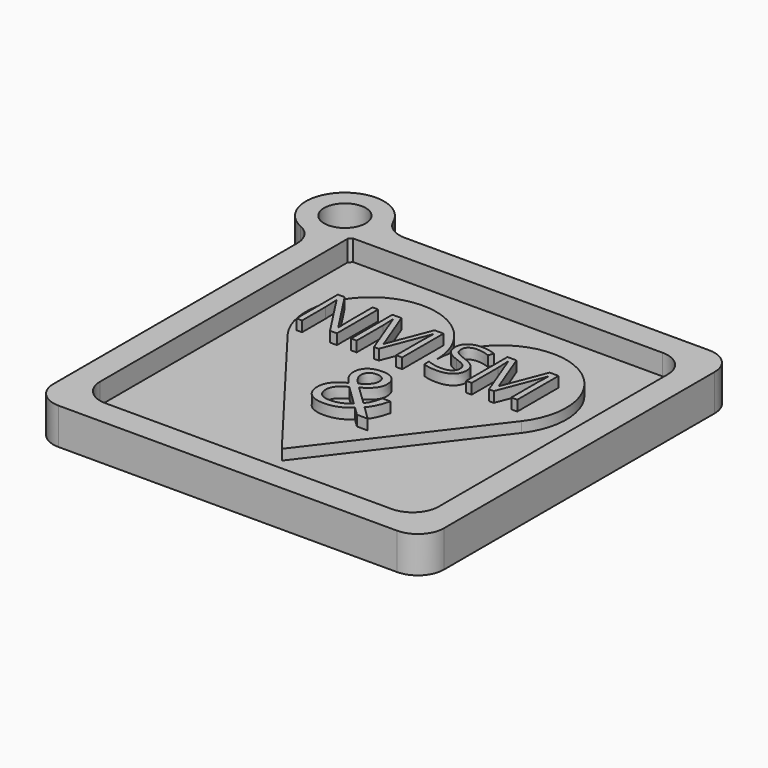
from build123d import *

# Parameters (mm, degrees)
F1_DEPTH       = 3
F2_DEPTH       = 5
F3_TEXT_SIZE   = 13.8888888889
F3_TEXT_SIZE_2 = 18.3928938996
F4_DEPTH       = 2
F5_DEPTH       = 2
F6_R           = 5


# Not quite as in the source:
# - a feature names something its author has since deleted; it is built from what else it names
# - Text() gives the source's letters only with a copy of the font that has no kerning and outlines rounded to 1/6400 em; it was checked with that copy


with BuildPart() as f1:
    # F0 (on Top) → F1 (new body)
    with BuildSketch(Plane.XY):
        with BuildLine():
            Line((32.5, 32.5), (-31.9098300563, 32.5))
            ThreePointArc((-31.9098300563, 32.5), (-32.1966991411, 32.1966991411), (-32.5, 31.9098300563))
            Line((-32.5, 31.9098300563), (-32.5, -32.5))
            Line((-32.5, -32.5), (32.5, -32.5))
            Line((32.5, -32.5), (32.5, 32.5))
        make_face()
        with BuildLine():
            ThreePointArc((-22.444038912, 4.925959459), (-16.4968433544, 24.3437850031), (0, 12.5))
            ThreePointArc((0, 12.5), (16.4968433544, 24.3437850031), (22.444038912, 4.925959459))
            Line((22.444038912, 4.925959459), (0, -24.5410595089))
            Line((0, -24.5410595089), (-22.444038912, 4.925959459))
        make_face(mode=Mode.SUBTRACT)
    extrude(amount=F1_DEPTH)

    # F0 (on Top) → F2 (join)
    with BuildSketch(Plane.XY):
        with BuildLine():
            ThreePointArc((-37.5, 33.5), (-40.3284271247, 40.3284271247), (-33.5, 37.5))
            Line((-33.5, 37.5), (-30, 37.5))
            ThreePointArc((-30, 37.5), (-42.8033008589, 42.8033008589), (-37.5, 30))
            Line((-37.5, 30), (-37.5, 33.5))
        make_face()
        with BuildLine():
            Line((-30, 37.5), (-33.5, 37.5))
            ThreePointArc((-33.5, 37.5), (-34.6715728753, 34.6715728753), (-37.5, 33.5))
            Line((-37.5, 33.5), (-37.5, 30))
            ThreePointArc((-37.5, 30), (-34.8238343267, 30.4937073078), (-32.5, 31.9098300563))
            Line((-32.5, 31.9098300563), (-32.5, 32.5))
            Line((-32.5, 32.5), (-31.9098300563, 32.5))
            ThreePointArc((-31.9098300563, 32.5), (-30.4937073078, 34.8238343267), (-30, 37.5))
        make_face()
        with BuildLine():
            Line((37.5, 37.5), (-30, 37.5))
            ThreePointArc((-30, 37.5), (-30.4937073078, 34.8238343267), (-31.9098300563, 32.5))
            Line((-31.9098300563, 32.5), (32.5, 32.5))
            Line((32.5, 32.5), (32.5, -32.5))
            Line((32.5, -32.5), (-32.5, -32.5))
            Line((-32.5, -32.5), (-32.5, 31.9098300563))
            ThreePointArc((-32.5, 31.9098300563), (-34.8238343267, 30.4937073078), (-37.5, 30))
            Line((-37.5, 30), (-37.5, -37.5))
            Line((-37.5, -37.5), (37.5, -37.5))
            Line((37.5, -37.5), (37.5, 37.5))
        make_face()
        with BuildLine():
            ThreePointArc((-32.5, 31.9098300563), (-32.1966991411, 32.1966991411), (-31.9098300563, 32.5))
            Line((-31.9098300563, 32.5), (-32.5, 32.5))
            Line((-32.5, 32.5), (-32.5, 31.9098300563))
        make_face()
        with BuildLine():
            ThreePointArc((22.444038912, 4.925959459), (16.4968433544, 24.3437850031), (0, 12.5))
            ThreePointArc((0, 12.5), (-16.4968433544, 24.3437850031), (-22.444038912, 4.925959459))
            Line((-22.444038912, 4.925959459), (0, -24.5410595089))
            Line((0, -24.5410595089), (22.444038912, 4.925959459))
        make_face()
    extrude(amount=F2_DEPTH)

    # F3 (on face) → F4 (join)
    with BuildSketch(Plane.XY.offset(5)):
        with Locations((-23.6911418243, 6.9181244482)):
            Text('NM', F3_TEXT_SIZE, font='Open Sans', text_align=(TextAlign.LEFT, TextAlign.BOTTOM))
        with Locations((1.2134523771, 6.9673178133)):
            Text('SM', F3_TEXT_SIZE, font='Open Sans', text_align=(TextAlign.LEFT, TextAlign.BOTTOM))
        with Locations((-7.0493952371, -11.8471132591)):
            Text('&', F3_TEXT_SIZE_2, font='Open Sans', text_align=(TextAlign.LEFT, TextAlign.BOTTOM))
    extrude(amount=F4_DEPTH)

    # F5 (add): a face of the model
    f5_faces = [f1.faces().sort_by_distance(p)[0] for p in [
        (-41.9783008589, 41.9783008589, 5),
    ]]
    extrude(f5_faces, amount=F5_DEPTH)

    # F6
    f6_edges = [f1.edges().sort_by_distance(p)[0] for p in [
        (-37.5, -37.5, 3.5),
        (37.5, -37.5, 3.5),
        (37.5, 37.5, 3.5),
        (-30, 37.5, 3.5),
        (-37.5, 30, 3.5),
        (32.5, 32.5, 5),
        (32.5, -32.5, 5),
        (-32.5, -32.5, 5),
    ]]
    fillet(f6_edges, radius=F6_R)


solid = f1.part
